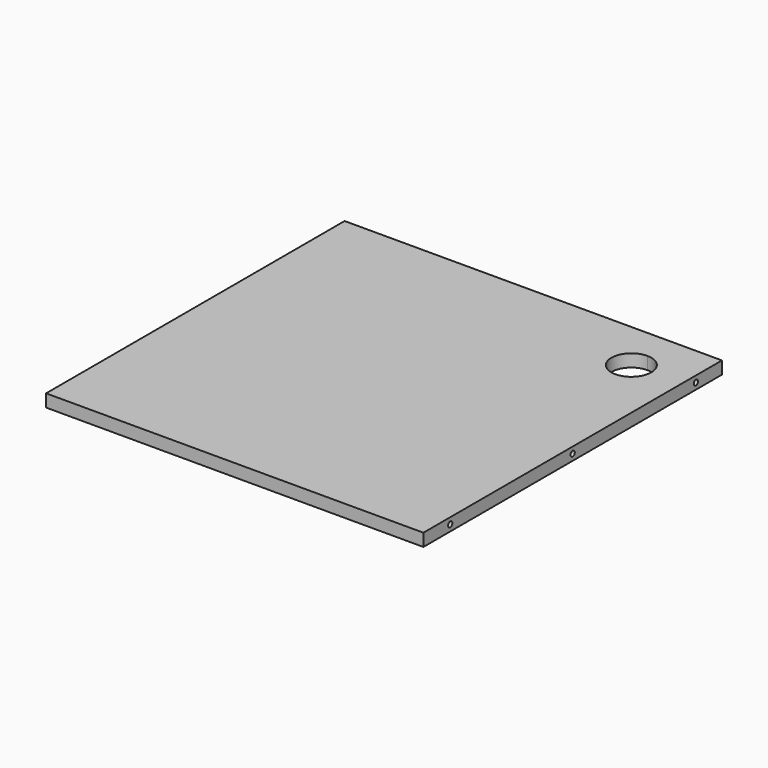
from build123d import *

# Parameters (mm, degrees)
F1_DEPTH = 19.05
F3_D     = 15.0114
F3_DEPTH = 14.224
F3_TIP   = 4.5098795482
F5_D     = 8.001
F5_DEPTH = 25.4
F5_TIP   = 2.4037429064
F7_D     = 8.001
F7_DEPTH = 25.4
F7_TIP   = 2.4037429064


# Not quite as in the source:
# - a feature names something its author has since deleted; it is built from what else it names


with BuildPart() as f1:
    # F0 (on Top) → F1 (new body)
    with BuildSketch(Plane.XY):
        with BuildLine():
            Line((209.55, 236.5375), (209.55, 282.575))
            Line((209.55, 282.575), (-285.75, 282.575))
            Line((-285.75, 282.575), (-285.75, -282.575))
            Line((-285.75, -282.575), (285.75, -282.575))
            Line((285.75, -282.575), (285.75, 206.375))
            Line((285.75, 206.375), (239.7125, 206.375))
            ThreePointArc((239.7125, 206.375), (188.2218917125, 185.0468917125), (209.55, 236.5375))
        make_face()
        with BuildLine():
            Line((285.75, 206.375), (285.75, 282.575))
            Line((285.75, 282.575), (209.55, 282.575))
            Line((209.55, 282.575), (209.55, 236.5375))
            ThreePointArc((209.55, 236.5375), (230.8781082875, 227.7031082875), (239.7125, 206.375))
            Line((239.7125, 206.375), (285.75, 206.375))
        make_face()
    extrude(amount=F1_DEPTH)

    # F3
    with Locations(Plane(origin=(0, 0, 0), x_dir=(1, 0, 0), z_dir=(0, 0, -1))):
        with Locations((-261.874, 231.775), (261.874, 231.775), (-261.874, 0), (261.874, 0), (261.874, -231.775), (-261.874, -231.775)):
            Hole(F3_D / 2, depth=F3_DEPTH)
            with Locations((0, 0, -(F3_DEPTH + F3_TIP / 2))):  # 118° drill point
                Cone(0, F3_D / 2, F3_TIP, mode=Mode.SUBTRACT)

    # F5
    with Locations(Plane.YZ.offset(285.75)):
        with Locations((-231.775, 9.525), (0, 9.525), (233.3625, 9.525)):
            Hole(F5_D / 2, depth=F5_DEPTH)
            with Locations((0, 0, -(F5_DEPTH + F5_TIP / 2))):  # 118° drill point
                Cone(0, F5_D / 2, F5_TIP, mode=Mode.SUBTRACT)

    # F7
    with Locations(Plane(origin=(-285.75, 0, 0), x_dir=(0, -1, 0), z_dir=(-1, 0, 0))):
        with Locations((0, 9.525), (231.775, 9.525), (-231.775, 9.525)):
            Hole(F7_D / 2, depth=F7_DEPTH)
            with Locations((0, 0, -(F7_DEPTH + F7_TIP / 2))):  # 118° drill point
                Cone(0, F7_D / 2, F7_TIP, mode=Mode.SUBTRACT)


solid = f1.part
